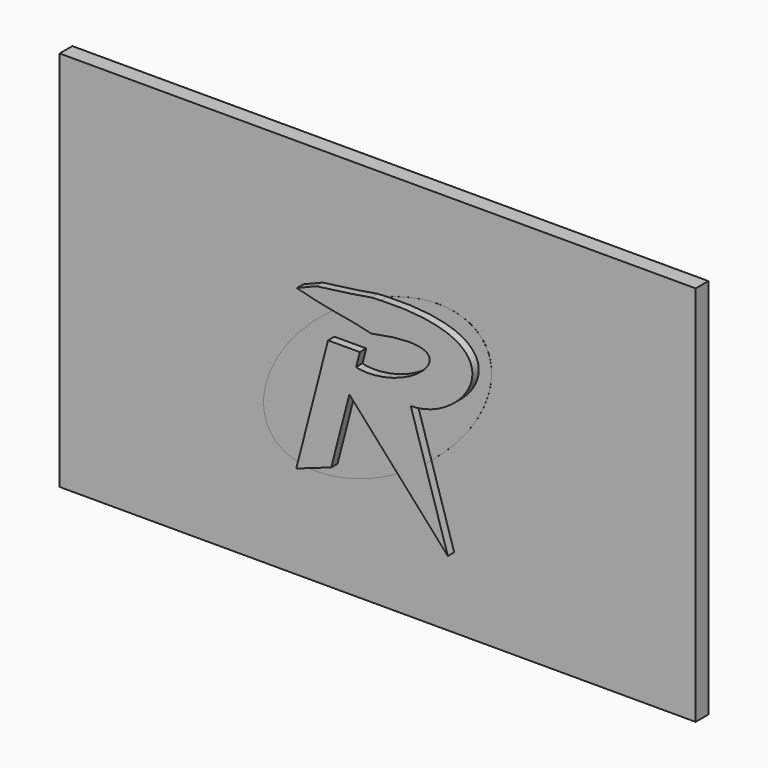
from build123d import *

# Parameters (mm, degrees)
F0_W     = 254
F0_H     = 152.4
F1_DEPTH = 6.35
F3_DEPTH = 0.0254
F5_DEPTH = 3.175


# Not quite as in the source:
# - a feature names something its author has since deleted; it is built from what else it names


with BuildPart() as f1:
    # F0 (on Front) → F1 (new body)
    with BuildSketch(Plane.XZ):
        Rectangle(F0_W, F0_H)
    extrude(amount=-F1_DEPTH)


with BuildPart() as f3:
    # F2 (on face) → F3 (new body)
    with BuildSketch(Plane.XZ):
        with BuildLine():
            add(Edge.make_bspline(
                [(42.7089780569, 29.5328665525), (15.3792632005, 69.0557550614), (-35.0193464566, 4.9950109782), (-85.4179561138, -59.0657331049), (-7.6896316003, -34.5278775307), (70.0386929133, -9.9900219565), (42.7089780569, 29.5328665525)],
                knots=[0, 0, 0, 2.0943951024, 2.0943951024, 4.1887902048, 4.1887902048, 6.2831853072, 6.2831853072, 6.2831853072], degree=2, weights=[1, 0.5, 1, 0.5, 1, 0.5, 1]))
        make_face()
    extrude(amount=F3_DEPTH)


with BuildPart() as f5:
    # F4 (on face) → F5 (new body)
    with BuildSketch(Plane.XZ.offset(0.0254)):
        with BuildLine():
            add(Edge.make_bspline(
                [(10.9512705407, -25.9492226202), (16.4828155374, -22.5918140848), (21.5058742199, -18.537459797)],
                knots=[4.6403572647, 4.6403572647, 4.6403572647, 4.8819348749, 4.8819348749, 4.8819348749], degree=2, weights=[0.8308791571, 0.7980759448, 0.7785771582]))
            Line((10.9512705407, -25.9492226202), (30.5927571669, -47.9500807992))
            Line((30.5927571669, -47.9500807992), (21.5058742199, -18.537459797))
        make_face()
        with BuildLine():
            Line((0, 33.02), (0, 31.6392348733))
            add(Edge.make_bspline(
                [(3.8851219863, 33.2129324059), (1.946109979, 32.4853248752), (0, 31.6392348733)],
                knots=[1.1236663731, 1.1236663731, 1.1236663731, 1.2014715695, 1.2014715695, 1.2014715695], degree=2, weights=[0.7513330658, 0.7526894283, 0.7554258571]))
            add(Edge.make_bspline(
                [(0, 33.02), (1.3337301063, 33.1020404773), (2.6284916435, 33.1661120443), (3.8851219863, 33.2129324059)],
                knots=[0, 0, 0, 0, 0.7676114314, 0.7676114314, 0.7676114314, 0.7676114314], degree=3))
        make_face()
        with BuildLine():
            Line((-8.7328994515, -3.9005538706), (10.9512705407, -25.9492226202))
            add(Edge.make_bspline(
                [(10.9512705407, -25.9492226202), (16.4828155374, -22.5918140848), (21.5058742199, -18.537459797)],
                knots=[4.6403572647, 4.6403572647, 4.6403572647, 4.8819348749, 4.8819348749, 4.8819348749], degree=2, weights=[0.8308791571, 0.7980759448, 0.7785771582]))
            Line((21.5058742199, -18.537459797), (15.7788182292, 0))
            add(Edge.make_bspline(
                [(3.8851219863, 33.2129324059), (62.53909114, 35.3983006502), (38.1200136526, 0), (15.7788182292, 0)],
                knots=[0.7676114314, 0.7676114314, 0.7676114314, 0.7676114314, 36.5963318477, 36.5963318477, 36.5963318477, 36.5963318477], degree=3))
            add(Edge.make_bspline(
                [(3.8851219863, 33.2129324059), (1.946109979, 32.4853248752), (0, 31.6392348733)],
                knots=[1.1236663731, 1.1236663731, 1.1236663731, 1.2014715695, 1.2014715695, 1.2014715695], degree=2, weights=[0.7513330658, 0.7526894283, 0.7554258571]))
            Line((0, 31.6392348733), (0, 20.32))
            add(Edge.make_bspline(
                [(0, 20.32), (42.7089780569, 29.5328665525), (17.9859120399, 3.6229274701), (-4.5411817708, 6.2032266552)],
                knots=[0, 0, 0, 0, 14.8292151358, 14.8292151358, 14.8292151358, 14.8292151358], degree=3))
            Line((-4.5411817708, 6.2032266552), (-6.0251812396, 6.5863936705))
            Line((-6.0251812396, 6.5863936705), (-8.7328994515, -3.9005538706))
        make_face()
        Polygon((-17.2411817708, 12.3338988988), (-29.9411817708, -36.852989598), (-15.9711817708, -31.9343007483), (-8.7328994515, -3.9005538706), (-6.0251812396, 6.5863936705), (-4.5411817708, 12.3338988988), align=None)
        with BuildLine():
            add(Edge.make_bspline(
                [(0, 31.6392348733), (-7.71435254, 28.2853460255), (-14.9981473119, 23.3527795901)],
                knots=[1.2014715695, 1.2014715695, 1.2014715695, 1.5155376104, 1.5155376104, 1.5155376104], degree=2, weights=[0.7554258571, 0.7664716411, 0.8000040736]))
            add(Edge.make_bspline(
                [(-14.9981473119, 23.3527795901), (-10.3762713203, 22.5418478133), (-6.2820866899, 21.9425380061), (0, 20.32)],
                knots=[14.0059934649, 14.0059934649, 14.0059934649, 14.0059934649, 30.3833855243, 30.3833855243, 30.3833855243, 30.3833855243], degree=3))
            Line((0, 20.32), (0, 31.6392348733))
        make_face()
        with BuildLine():
            add(Edge.make_bspline(
                [(-29.7124151815, 26.67), (-23.2893696753, 24.8945764216), (-18.9507891427, 24.0462908112), (-14.9981473119, 23.3527795901)],
                knots=[0, 0, 0, 0, 14.0059934649, 14.0059934649, 14.0059934649, 14.0059934649], degree=3))
            add(Edge.make_bspline(
                [(0, 31.6392348733), (-7.71435254, 28.2853460255), (-14.9981473119, 23.3527795901)],
                knots=[1.2014715695, 1.2014715695, 1.2014715695, 1.5155376104, 1.5155376104, 1.5155376104], degree=2, weights=[0.7554258571, 0.7664716411, 0.8000040736]))
            Line((0, 31.6392348733), (0, 33.02))
            add(Edge.make_bspline(
                [(-21.8985817649, 29.845), (-9.461321868, 31.493146081), (-6.9059981033, 31.7937714201), (0, 33.02)],
                knots=[0, 0, 0, 0, 22.1275508883, 22.1275508883, 22.1275508883, 22.1275508883], degree=3))
            Line((-21.8985817649, 29.845), (-29.7124151815, 26.67))
        make_face()
    extrude(amount=F5_DEPTH)


solid = Compound([f1.part, f3.part, f5.part])
